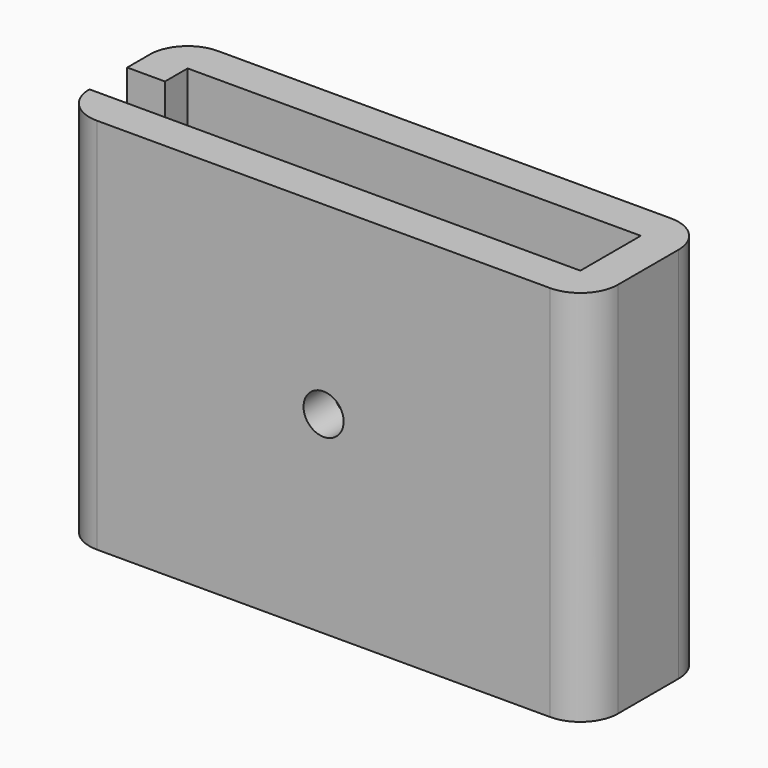
from build123d import *

# Parameters (mm, degrees)
F1_DEPTH = 50.8
F2_R     = 5.07999
F3_R     = 2.6971074435
F4_DEPTH = 25.4


# Not quite as in the source:
# - a fillet or chamfer is up to 0.001 mm smaller than in the source, because OpenCascade refuses the exact size


with BuildPart() as f1:
    # F0 (on Top) → F1 (new body)
    with BuildSketch(Plane.XY):
        Polygon((-30.48, 1.27), (-30.48, 5.08), (30.48, 5.08), (30.48, -5.08), (-30.48, -5.08), (-35.56, -5.08), (-35.56, -10.16), (35.56, -10.16), (35.56, 10.16), (-35.56, 10.16), (-35.56, 1.27), align=None)
    extrude(amount=F1_DEPTH)

    # F2 (radius 5.08 in the source; OpenCascade refuses exactly that, so slightly less here)
    f2_edges = [f1.edges().sort_by_distance(p)[0] for p in [
        (35.56, 10.16, 25.4),
        (35.56, -10.16, 25.4),
        (-35.56, 10.16, 25.4),
        (-35.56, -10.16, 25.4),
    ]]
    fillet(f2_edges, radius=F2_R)

    # F3 (on face) → F4 (cut)
    with BuildSketch(Plane.XZ.offset(10.16)):
        with Locations((0, 25.9590707719)):
            Circle(F3_R)
    extrude(amount=-F4_DEPTH, mode=Mode.SUBTRACT)


solid = f1.part
